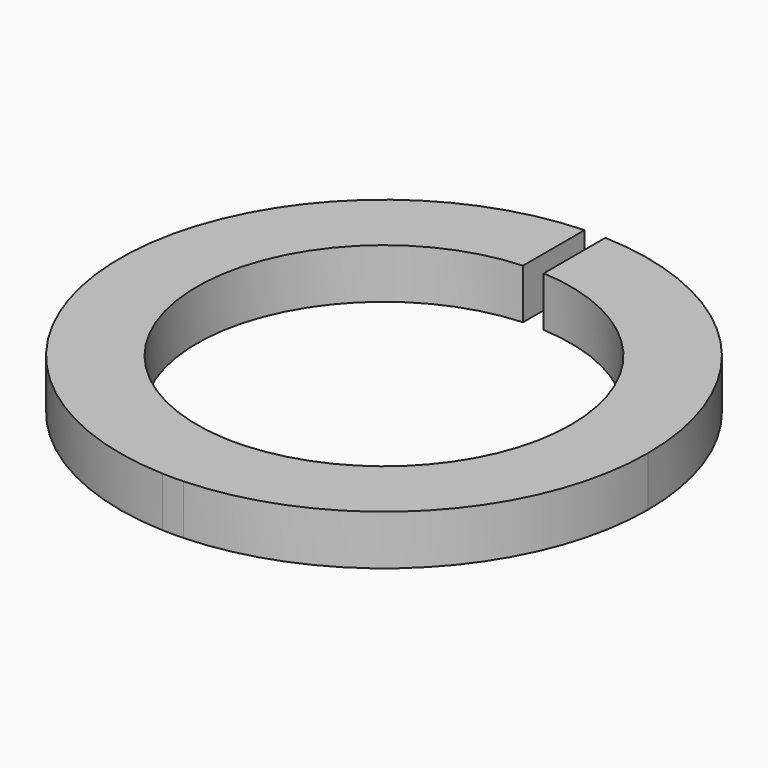
from build123d import *

# Parameters (mm, degrees)
F1_DEPTH = 1.524


# Not quite as in the source:
# - a feature names something its author has since deleted; it is built from what else it names


with BuildPart() as f1:
    # F0 (on Top) → F1 (new body)
    with BuildSketch(Plane.XY):
        with BuildLine():
            ThreePointArc((0.3175, 5.7061737399), (4.1518512437, 3.9272581084), (5.715, 0))
            ThreePointArc((5.715, 0), (4.1518512437, -3.9272581084), (0.3175, -5.7061737399))
            Line((0.3175, -5.7061737399), (0.3175, -8.0582475762))
            ThreePointArc((0.3175, -8.0582475762), (5.8136322123, -5.5890822816), (8.0645, 0))
            ThreePointArc((8.0645, 0), (5.8136322123, 5.5890822816), (0.3175, 8.0582475762))
            Line((0.3175, 8.0582475762), (0.3175, 5.7061737399))
        make_face()
        with BuildLine():
            Line((0.3175, -8.0582475762), (0.3175, -5.7061737399))
            ThreePointArc((0.3175, -5.7061737399), (0, -5.715), (-0.3175, -5.7061737399))
            Line((-0.3175, -5.7061737399), (-0.3175, -8.0582475762))
            ThreePointArc((-0.3175, -8.0582475762), (0, -8.0645), (0.3175, -8.0582475762))
        make_face()
        with BuildLine():
            ThreePointArc((-0.3175, -5.7061737399), (-5.715, 0), (-0.3175, 5.7061737399))
            Line((-0.3175, 5.7061737399), (-0.3175, 8.0582475762))
            ThreePointArc((-0.3175, 8.0582475762), (-8.0645, 0), (-0.3175, -8.0582475762))
            Line((-0.3175, -8.0582475762), (-0.3175, -5.7061737399))
        make_face()
    extrude(amount=F1_DEPTH)


solid = f1.part
